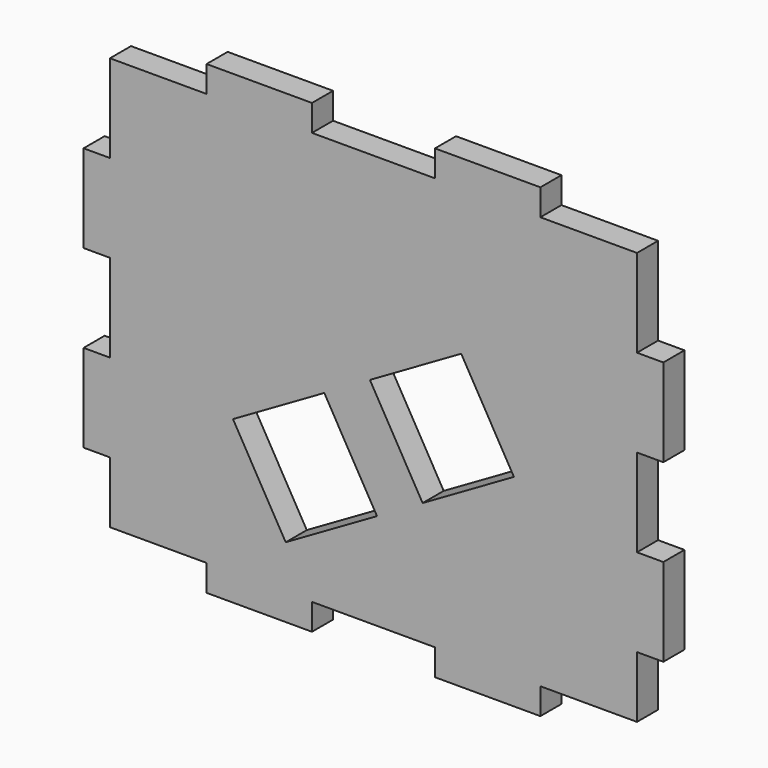
from build123d import *

# Parameters (mm, degrees)
F1_DEPTH = 3


# Not quite as in the source:
# - a feature names something its author has since deleted; it is built from what else it names


with BuildPart() as f1:
    # F0 (on Front) → F1 (new body)
    with BuildSketch(Plane.XZ):
        Polygon((-19, 26.5), (-19, 23.5), (-30, 23.5), (-30, 13.5), (-33, 13.5), (-33, 3.5), (-30, 3.5), (-30, -6.5), (-33, -6.5), (-33, -16.5), (-30, -16.5), (-30, -23.5), (-19, -23.5), (-19, -26.5), (-7, -26.5), (-7, -23.5), (7, -23.5), (7, -26.5), (19, -26.5), (19, -23.5), (30, -23.5), (30, -16.5), (33, -16.5), (33, -6.5), (30, -6.5), (30, 3.5), (33, 3.5), (33, 13.5), (30, 13.5), (30, 23.5), (19, 23.5), (19, 26.5), (7, 26.5), (7, 23.5), (-7, 23.5), (-7, 26.5), align=None)
        Polygon((0.4019237886, -12.5), (-9.9903810568, -18.5), (-15.9903810568, -8.1076951546), (-5.5980762114, -2.1076951546), align=None, mode=Mode.SUBTRACT)
        Polygon((-0.4019237886, 0.8923048454), (9.9903810568, 6.8923048454), (15.9903810568, -3.5), (5.5980762114, -9.5), align=None, mode=Mode.SUBTRACT)
    extrude(amount=F1_DEPTH)


solid = f1.part
